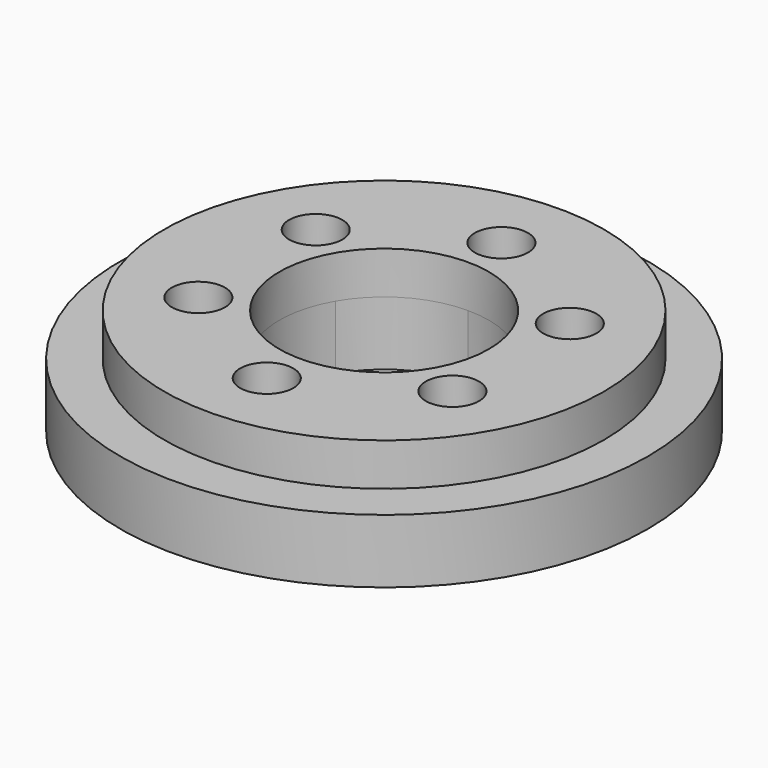
from build123d import *
from build123d import SkipClean  # not in build123d's __all__

# Parameters (mm, degrees)
F0_R     = 31.496
F1_DEPTH = 7.62
F2_R     = 26.2255
F2_R_2   = 3.175
F2_R_3   = 12.4968
F3_DEPTH = 5.08


with BuildPart() as f1:
    # F0 (on Top) → F1 (new body)
    with BuildSketch(Plane.XY):
        Circle(F0_R)
        with BuildLine():
            ThreePointArc((-11.9809641815, -8.7503), (-18.2227786799, -9.5720504682), (-12.4063335245, -7.1628))
            ThreePointArc((-12.4063335245, -7.1628), (-12.089149683, -7.9285495318), (-11.9809641815, -8.7503))
        make_face(mode=Mode.SUBTRACT)
        with BuildLine():
            ThreePointArc((3.175, -17.5006), (-2.2450640303, -19.7456640303), (0, -14.3256))
            ThreePointArc((0, -14.3256), (2.2450640303, -15.2555359697), (3.175, -17.5006))
        make_face(mode=Mode.SUBTRACT)
        with BuildLine():
            ThreePointArc((18.3309641815, -8.7503), (14.3342137133, -11.8171144985), (12.4063335245, -7.1628))
            ThreePointArc((12.4063335245, -7.1628), (15.9777146497, -5.6834855015), (18.3309641815, -8.7503))
        make_face(mode=Mode.SUBTRACT)
        with BuildLine():
            ThreePointArc((-11.9809641815, 8.7503), (-12.089149683, 7.9285495318), (-12.4063335245, 7.1628))
            ThreePointArc((-12.4063335245, 7.1628), (-18.2227786799, 9.5720504682), (-11.9809641815, 8.7503))
        make_face(mode=Mode.SUBTRACT)
        with BuildLine():
            ThreePointArc((10.822546266, 6.2484), (12.070981866, 3.2344098428), (12.4968, 0))
            ThreePointArc((12.4968, 0), (12.070981866, -3.2344098428), (10.822546266, -6.2484))
            ThreePointArc((10.822546266, -6.2484), (6.2484, -10.822546266), (0, -12.4968))
            ThreePointArc((0, -12.4968), (-6.2484, -10.822546266), (-10.822546266, -6.2484))
            ThreePointArc((-10.822546266, -6.2484), (-12.4968, 0), (-10.822546266, 6.2484))
            ThreePointArc((-10.822546266, 6.2484), (-6.2484, 10.822546266), (0, 12.4968))
            ThreePointArc((0, 12.4968), (6.2484, 10.822546266), (10.822546266, 6.2484))
        make_face(mode=Mode.SUBTRACT)
        with BuildLine():
            ThreePointArc((18.3309641815, 8.7503), (15.9777146497, 5.6834855015), (12.4063335245, 7.1628))
            ThreePointArc((12.4063335245, 7.1628), (14.3342137133, 11.8171144985), (18.3309641815, 8.7503))
        make_face(mode=Mode.SUBTRACT)
        with BuildLine():
            ThreePointArc((3.175, 17.5006), (2.2450640303, 15.2555359697), (0, 14.3256))
            ThreePointArc((0, 14.3256), (-2.2450640303, 19.7456640303), (3.175, 17.5006))
        make_face(mode=Mode.SUBTRACT)
    extrude(amount=F1_DEPTH)

    # F2 (on face) → F3 (join)
    with BuildSketch(Plane.XY.offset(7.62)):
        Circle(F2_R)
        with Locations((-15.1559641815, -8.7503)):
            Circle(F2_R_2, mode=Mode.SUBTRACT)
        with Locations((0, -17.5006)):
            Circle(F2_R_2, mode=Mode.SUBTRACT)
        with Locations((15.1559641815, -8.7503)):
            Circle(F2_R_2, mode=Mode.SUBTRACT)
        with Locations((-15.1559641815, 8.7503)):
            Circle(F2_R_2, mode=Mode.SUBTRACT)
        Circle(F2_R_3, mode=Mode.SUBTRACT)
        with Locations((15.1559641815, 8.7503)):
            Circle(F2_R_2, mode=Mode.SUBTRACT)
        with Locations((0, 17.5006)):
            Circle(F2_R_2, mode=Mode.SUBTRACT)
    with SkipClean():  # cleaning this boolean's faces spoils the solid; the shape is the same uncleaned
        extrude(amount=F3_DEPTH)


solid = f1.part
